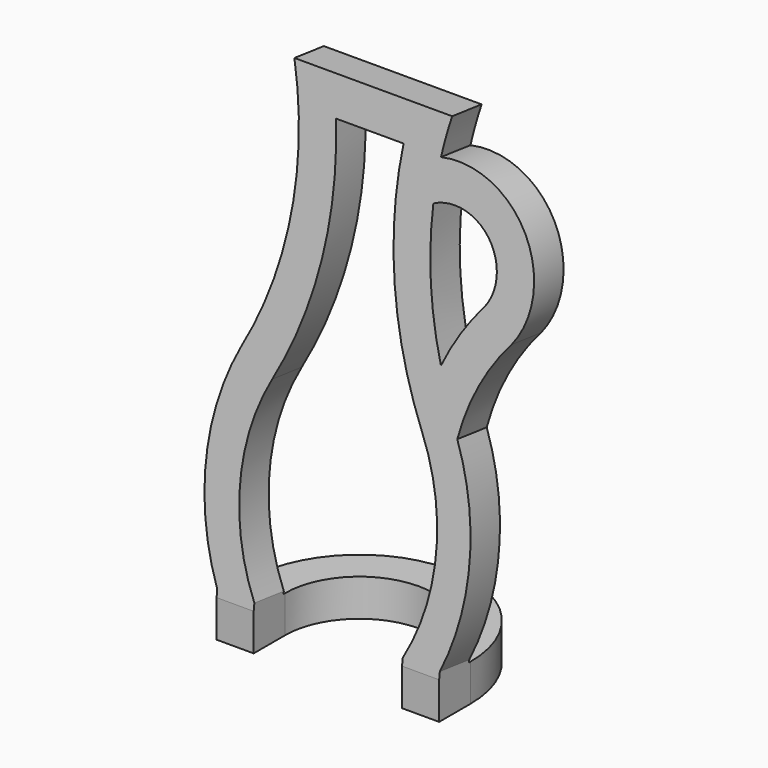
from build123d import *

# Parameters (mm, degrees)
F4_DEPTH = 25.4
F6_DEPTH = 25.4


# Not quite as in the source:
# - ends of sketch curves that miss each other by under 0.0002 mm in the source are joined


with BuildPart() as f4:
    # F3 (on offset) → F4 (new body)
    with BuildSketch(Plane.XY):
        with BuildLine():
            Line((-76.2, 26.9875), (-76.2, 0))
            Line((-76.2, 0), (-50.8, 0))
            Line((-50.8, 0), (-50.8, 26.9875))
            ThreePointArc((-50.8, 26.9875), (0, 77.7875), (50.8, 26.9875))
            Line((50.8, 26.9875), (50.8, 0))
            Line((50.8, 0), (76.2, 0))
            Line((76.2, 0), (76.2, 26.9875))
            ThreePointArc((76.2, 26.9875), (0, 103.1875), (-76.2, 26.9875))
        make_face()
    extrude(amount=-F4_DEPTH)

    # F5 (on line) → F6 (join)
    with BuildSketch(Plane(origin=(0, 0, 0), x_dir=(-1, 0, 0), z_dir=(0, 0.9925461516, -0.1218693434))):
        with BuildLine():
            ThreePointArc((-75.0903723478, 138.827645489), (-90.0403532632, 71.9142183688), (-76.2, 4.7625))
            Line((-76.2, 4.7625), (-76.2, 0))
            Line((-76.2, 0), (-50.8, 0))
            Line((-50.8, 0), (-50.8, 4.7625))
            ThreePointArc((-50.8, 4.7625), (-67.302415347, 70.0192610552), (-51.3729695475, 135.4182467678))
            ThreePointArc((-51.3729695475, 135.4182467678), (-25.0838158912, 212.3805783338), (-23.2117561056, 293.6875002493))
            Line((-23.2117561056, 293.6875002493), (0, 293.6875002493))
            Line((0, 293.6875002493), (23.1415493167, 293.6875002493))
            ThreePointArc((23.1415493167, 293.6875002493), (24.7523028396, 211.7684987185), (51.1552849917, 134.2043325579))
            ThreePointArc((51.1552849917, 134.2043325579), (66.8742650231, 69.439784083), (50.8, 4.7625))
            Line((50.8, 4.7625), (50.8, 0))
            Line((50.8, 0), (76.2, 0))
            Line((76.2, 0), (76.2, 4.7625))
            ThreePointArc((76.2, 4.7625), (90.7935935425, 75.6597014149), (73.6577047551, 145.9857098073))
            ThreePointArc((73.6577047551, 145.9857098073), (47.6694306232, 230.702066542), (54.0150973414, 319.0874952316))
            Line((54.0150973414, 319.0874952316), (0, 319.0874952316))
            Line((0, 319.0874952316), (-54.0150973414, 319.0874952316))
            ThreePointArc((-54.0150973414, 319.0874952316), (-51.0804025225, 306.5319685143), (-48.8205663921, 293.8376065574))
            ThreePointArc((-48.8205663921, 293.8376065574), (-108.938602772, 268.4421399471), (-106.0506710111, 203.2442268465))
            ThreePointArc((-106.0506710111, 203.2442268465), (-86.3813942483, 173.049340693), (-75.0903723478, 138.827645489))
        make_face()
        with BuildLine():
            ThreePointArc((-46.2746955842, 266.2427872527), (-48.9959426673, 220.834025793), (-60.1912430767, 176.7429149913))
            ThreePointArc((-60.1912430767, 176.7429149913), (-71.5917023099, 198.9100774911), (-86.1994937771, 219.1082455385))
            ThreePointArc((-86.1994937771, 219.1082455385), (-84.8490348444, 258.4405568096), (-46.2746955842, 266.2427872527))
        make_face(mode=Mode.SUBTRACT)
    extrude(amount=F6_DEPTH)


solid = f4.part
